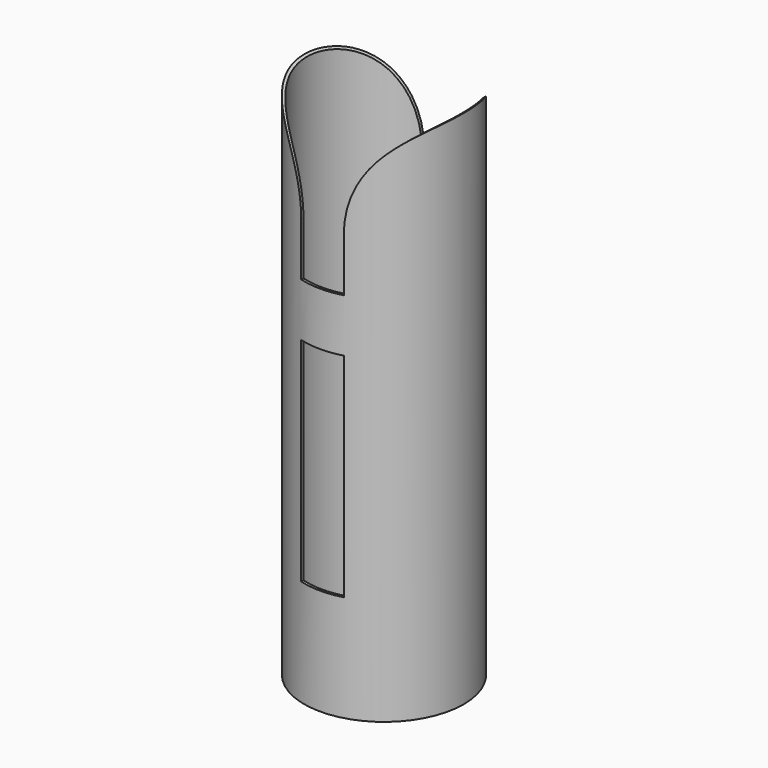
from build123d import *

# Parameters (mm, degrees)
F0_R        = 19.05
F1_DEPTH    = 127
F2_T        = -0.635
F3_W        = 10.16
F3_H        = 50.8
F3_H_2      = 127
F4_DEPTH    = 38.1
F5_T1_DEPTH = 127.6597299865
F5_T3_DEPTH = 127.6597299858
F5_T5_DEPTH = 127.6597299858
F5_T7_DEPTH = 127.6597299865


# Not quite as in the source:
# - a fillet or chamfer that OpenCascade refuses, or shapes differently, is made with other operations: its cross-section is extruded or revolved along the edge and cut away or added


with BuildPart() as f1:
    # F0 (on Top) → F1 (new body)
    with BuildSketch(Plane.XY):
        Circle(F0_R)
    extrude(amount=F1_DEPTH)

    # F2
    f2_openings = [f1.faces().sort_by_distance(p)[0] for p in [
        (0, 0, 0),
        (0, 0, 127),
    ]]
    offset(amount=F2_T, openings=f2_openings)

    # F3 (on Front) → F4 (cut, symmetric)
    with BuildSketch(Plane.XZ):
        with Locations((0, 50.8)):
            Rectangle(F3_W, F3_H)
        with Locations((-3.17e-08, 114.3)):
            Rectangle(F3_W, F3_H)
        with Locations((-0.4444076066, 213.36)):
            Rectangle(F3_W, F3_H_2)
    extrude(amount=F4_DEPTH, both=True, mode=Mode.SUBTRACT)

    # F5: fillet of radius 25.4 on 4 edges, made by hand

    # F5_s2 → F5_t1 (cut)
    with BuildSketch(Plane.XZ.offset(-45.7995529809)):
        with BuildLine():
            ThreePointArc((-5.0800000317, 101.6), (-12.5194877896, 119.5605122421), (-30.4800000317, 127))
            Line((-30.4800000317, 127), (-5.0800000317, 127))
            Line((-5.0800000317, 127), (-5.0800000317, 101.6))
        make_face()
    extrude(amount=F5_T1_DEPTH, mode=Mode.SUBTRACT)

    # F5_s4 → F5_t3 (cut)
    with BuildSketch(Plane.XZ.offset(-45.7995529626)):
        with BuildLine():
            ThreePointArc((30.4799999683, 127), (12.5194877261, 119.5605122421), (5.0799999683, 101.6))
            Line((5.0799999683, 101.6), (5.0799999683, 127))
            Line((5.0799999683, 127), (30.4799999683, 127))
        make_face()
    extrude(amount=F5_T3_DEPTH, mode=Mode.SUBTRACT)

    # F5_s6 → F5_t5 (cut)
    with BuildSketch(Plane.XZ.offset(-81.8601770232)):
        with BuildLine():
            ThreePointArc((30.4799999683, 127), (12.5194877261, 119.5605122421), (5.0799999683, 101.6))
            Line((5.0799999683, 101.6), (5.0799999683, 127))
            Line((5.0799999683, 127), (30.4799999683, 127))
        make_face()
    extrude(amount=F5_T5_DEPTH, mode=Mode.SUBTRACT)

    # F5_s8 → F5_t7 (cut)
    with BuildSketch(Plane.XZ.offset(-81.8601770056)):
        with BuildLine():
            ThreePointArc((-30.4800000317, 127), (-12.5194877896, 119.5605122421), (-5.0800000317, 101.6))
            Line((-5.0800000317, 101.6), (-5.0800000317, 127))
            Line((-5.0800000317, 127), (-30.4800000317, 127))
        make_face()
    extrude(amount=F5_T7_DEPTH, mode=Mode.SUBTRACT)


solid = f1.part
